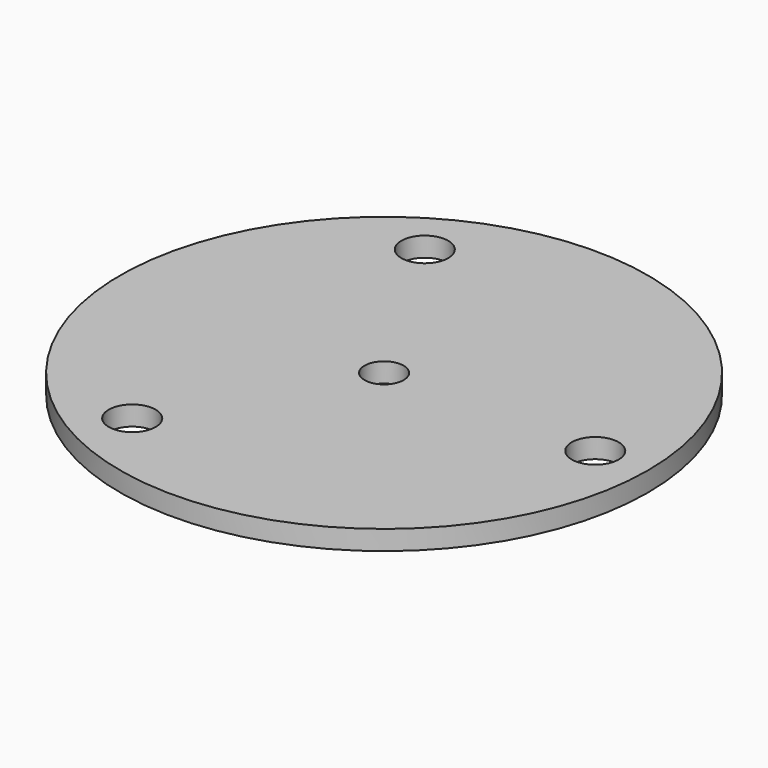
from build123d import *

# Parameters (mm, degrees)
F0_R            = 67.5
F0_R_2          = 5
F1_DEPTH        = 5
F3_D            = 12
F3_COPIES_COUNT = 3


# Not quite as in the source:
# - a pattern or mirror of a feature is missing from the dataset's text; its kind, count and spacing are read off the source's solid


with BuildPart() as f1:
    # F0 (on Top) → F1 (new body)
    with BuildSketch(Plane.XY):
        Circle(F0_R)
        Circle(F0_R_2, mode=Mode.SUBTRACT)
    extrude(amount=F1_DEPTH)

    # F3 (through all)
    with Locations(Plane.XY.offset(5)):
        with Locations((54, 0)):
            f3 = Hole(F3_D / 2)

    # F3_copies: F3 ×3 about axis
    f3_copies_axis = Axis((0, 0, 0), (0, 0, 1))
    for i in range(1, F3_COPIES_COUNT):
        add(f3.rotate(f3_copies_axis, i * 360 / F3_COPIES_COUNT), mode=Mode.SUBTRACT)


solid = f1.part
